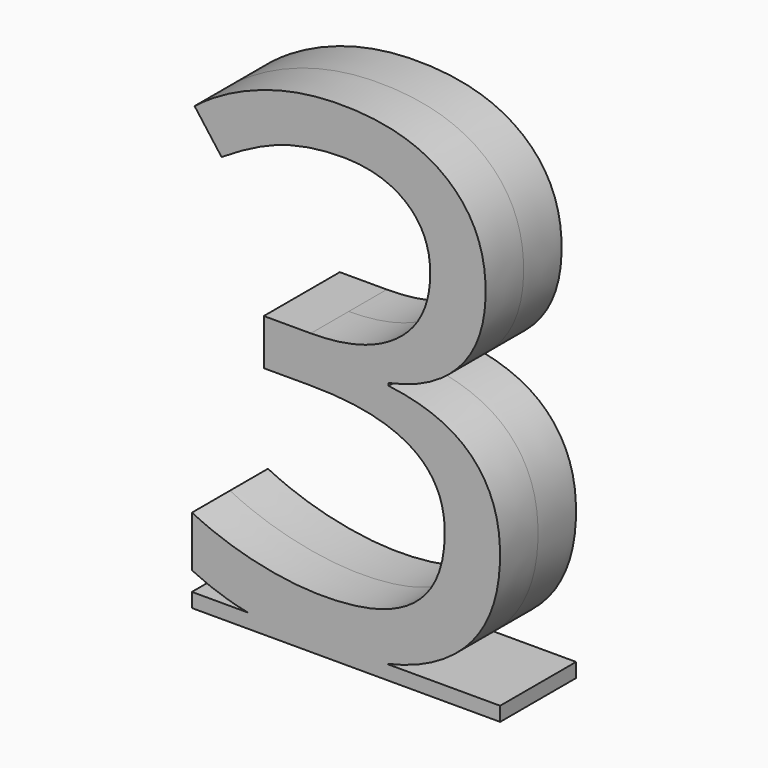
from build123d import *

# Parameters (mm, degrees)
F0_TEXT_SIZE  = 138.8888888889
F1_DEPTH      = 10
F1_DEPTH_BACK = 10
F2_W          = 64.919343094
F2_H          = 20
F3_DEPTH      = 3


# Not quite as in the source:
# - Text() gives the source's letters only with a copy of the font that has no kerning and outlines rounded to 1/6400 em; it was checked with that copy


with BuildPart() as f1:
    # F0 (on Front) → F1 (new body, two sides)
    with BuildSketch(Plane.XZ) as f1_sk:
        with Locations((-40.13671875, 0)):
            Text('3', F0_TEXT_SIZE, font='Open Sans', text_align=(TextAlign.LEFT, TextAlign.BOTTOM))
    extrude(amount=F1_DEPTH)
    extrude(f1_sk.sketch, amount=-F1_DEPTH_BACK)

    # F2 (on Top) → F3 (join)
    with BuildSketch(Plane.XY):
        with Locations((-1.317604714, 0)):
            Rectangle(F2_W, F2_H)
    extrude(amount=-F3_DEPTH)


solid = f1.part
